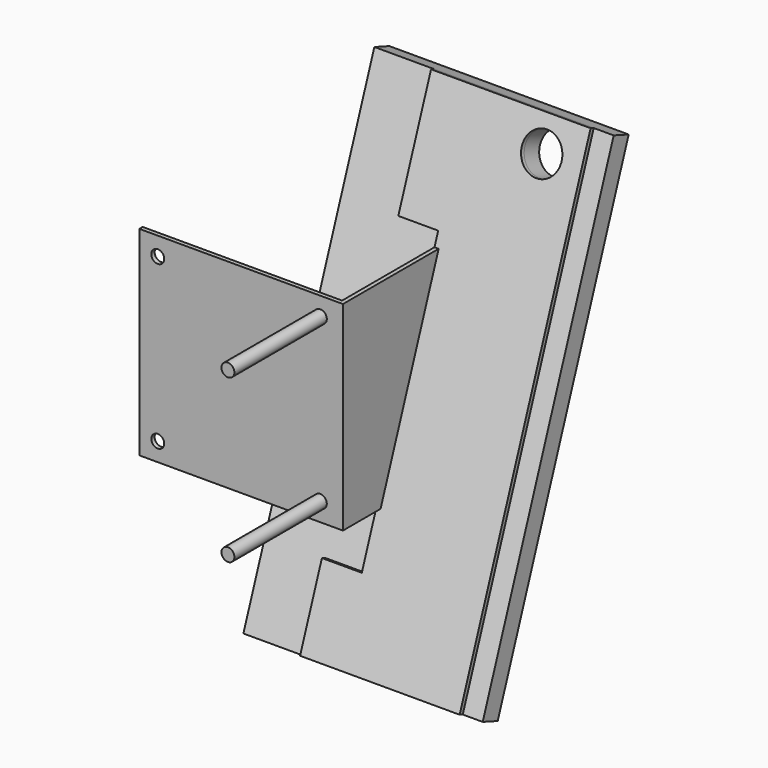
from build123d import *

# Parameters (mm, degrees)
F0_R      = 4.1275
F1_DEPTH  = 2.65684
F4_DEPTH  = 2.65684
F5_R      = 6.35
F5_R_2    = 4.1275
F6_DEPTH  = 6.35
F7_DEPTH  = 76.2
F8_R      = 12.7
F8_W      = 25.4
F8_H      = 76.2
F8_H_2    = 50.8
F9_DEPTH  = 2.65684
F10_W     = 152.4
F10_H     = 304.8
F10_R     = 12.7
F11_DEPTH = 12.7


with BuildPart() as f1:
    # F0 (on Front) → F1 (new body)
    with BuildSketch(Plane.XZ):
        with BuildLine():
            Line((47.625, -47.625), (46.9269177812, -47.625))
            ThreePointArc((46.9269177812, -47.625), (49.5524939874, -57.7092166749), (58.1025, -51.7525))
            ThreePointArc((58.1025, -51.7525), (54.4088955842, -45.9848260754), (47.625, -46.9269177812))
            Line((47.625, -46.9269177812), (47.625, -47.625))
        make_face()
        with Locations((51.7525, -51.7525)):
            Circle(F0_R, mode=Mode.SUBTRACT)
        with BuildLine():
            Line((46.9269177812, 47.625), (0, 47.625))
            Line((0, 47.625), (0, -47.625))
            Line((0, -47.625), (46.9269177812, -47.625))
            ThreePointArc((46.9269177812, -47.625), (47.2623719395, -47.2623719395), (47.625, -46.9269177812))
            Line((47.625, -46.9269177812), (47.625, 46.9269177812))
            ThreePointArc((47.625, 46.9269177812), (47.2623719395, 47.2623719395), (46.9269177812, 47.625))
        make_face()
        with BuildLine():
            Line((63.5, 63.5), (0, 63.5))
            Line((0, 63.5), (0, 47.625))
            Line((0, 47.625), (46.9269177812, 47.625))
            ThreePointArc((46.9269177812, 47.625), (49.5524939874, 57.7092166749), (58.1025, 51.7525))
            ThreePointArc((58.1025, 51.7525), (54.4088955842, 45.9848260754), (47.625, 46.9269177812))
            Line((47.625, 46.9269177812), (47.625, -46.9269177812))
            ThreePointArc((47.625, -46.9269177812), (54.4088955842, -45.9848260754), (58.1025, -51.7525))
            ThreePointArc((58.1025, -51.7525), (49.5524939874, -57.7092166749), (46.9269177812, -47.625))
            Line((46.9269177812, -47.625), (0, -47.625))
            Line((0, -47.625), (0, -63.5))
            Line((0, -63.5), (63.5, -63.5))
            Line((63.5, -63.5), (63.5, 63.5))
        make_face()
        with BuildLine():
            ThreePointArc((58.1025, 51.7525), (49.5524939874, 57.7092166749), (46.9269177812, 47.625))
            Line((46.9269177812, 47.625), (47.625, 47.625))
            Line((47.625, 47.625), (47.625, 46.9269177812))
            ThreePointArc((47.625, 46.9269177812), (54.4088955842, 45.9848260754), (58.1025, 51.7525))
        make_face()
        with Locations((51.7525, 51.7525)):
            Circle(F0_R, mode=Mode.SUBTRACT)
        with BuildLine():
            Line((47.625, 47.625), (46.9269177812, 47.625))
            ThreePointArc((46.9269177812, 47.625), (47.2623719395, 47.2623719395), (47.625, 46.9269177812))
            Line((47.625, 46.9269177812), (47.625, 47.625))
        make_face()
        with BuildLine():
            ThreePointArc((47.625, -46.9269177812), (47.2623719395, -47.2623719395), (46.9269177812, -47.625))
            Line((46.9269177812, -47.625), (47.625, -47.625))
            Line((47.625, -47.625), (47.625, -46.9269177812))
        make_face()
    extrude(amount=F1_DEPTH)

    # F2: F1 across plane


with BuildPart() as f1_1:
    add(f1.part)
    add(f1.part.mirror(Plane.YZ))

    # F3 (on face) → F4 (join)
    with BuildSketch(Plane.YZ.offset(63.5)):
        Polygon((-2.65684, 63.5), (-2.65684, -63.5), (27.3189402482, -63.5), (73.54316, 63.5), align=None)
    extrude(amount=F4_DEPTH)

    # F8 (on face) + F5 (on face) → F9 (join)
    with BuildSketch(Plane(origin=(0, 44.5317379162, -16.2082270816), x_dir=(-1, 0, 0), z_dir=(0, 0.9396926208, -0.3420201433))):
        Polygon((-63.5, 169.6484349915), (-139.7, 169.6484349915), (-139.7, -135.1515650085), (-63.5, -135.1515650085), (-63.5, -84.3515650085), (-63.5, 93.4484349915), align=None)
        with Locations((-114.3, 148.6934349915)):
            Circle(F8_R, mode=Mode.SUBTRACT)
        with Locations((-50.8, 131.5484349915)):
            Rectangle(F8_W, F8_H)
        with Locations((-50.8, -109.7515650085)):
            Rectangle(F8_W, F8_H_2)
    with BuildSketch(Plane(origin=(0, 0, 0), x_dir=(-1, 0, 0), z_dir=(0, 1, 0))):
        with Locations((-51.7525, 51.7525)):
            Circle(F5_R)
        with Locations((-51.7525, -51.7525)):
            Circle(F5_R)
    extrude(amount=F9_DEPTH, dir=(0, 0.9396926208, -0.3420201433))


with BuildPart() as f6:
    # F5 (on face) → F6 (new body)
    with BuildSketch(Plane(origin=(0, 0, 0), x_dir=(-1, 0, 0), z_dir=(0, 1, 0))):
        with Locations((-51.7525, 51.7525)):
            Circle(F5_R)
        with Locations((-51.7525, 51.7525)):
            Circle(F5_R_2, mode=Mode.SUBTRACT)
        with Locations((-51.7525, 51.7525)):
            Circle(F5_R_2)
    extrude(amount=F6_DEPTH)

    # F5 (on face) → F7, piece 2 (join)
    with BuildSketch(Plane(origin=(0, 0, 0), x_dir=(-1, 0, 0), z_dir=(0, 1, 0))):
        with Locations((-51.7525, 51.7525)):
            Circle(F5_R_2)
    extrude(amount=-F7_DEPTH)


with BuildPart() as f6b:
    # F5 (on face) → F6, piece 2 (new body)
    with BuildSketch(Plane(origin=(0, 0, 0), x_dir=(-1, 0, 0), z_dir=(0, 1, 0))):
        with Locations((-51.7525, -51.7525)):
            Circle(F5_R)
        with Locations((-51.7525, -51.7525)):
            Circle(F5_R_2, mode=Mode.SUBTRACT)
        with Locations((-51.7525, -51.7525)):
            Circle(F5_R_2)
    extrude(amount=F6_DEPTH)

    # F5 (on face) → F7 (join)
    with BuildSketch(Plane(origin=(0, 0, 0), x_dir=(-1, 0, 0), z_dir=(0, 1, 0))):
        with Locations((-51.7525, -51.7525)):
            Circle(F5_R_2)
    extrude(amount=-F7_DEPTH)


with BuildPart() as f11:
    # F10 (on face) → F11 (new body)
    with BuildSketch(Plane(origin=(0, 47.0283508588, -17.1169198792), x_dir=(-1, 0, 0), z_dir=(0, 0.9396926208, -0.3420201433))):
        with Locations((-76.2, 17.2484349915)):
            Rectangle(F10_W, F10_H)
        with Locations((-114.3, 148.6934349915)):
            Circle(F10_R, mode=Mode.SUBTRACT)
    extrude(amount=F11_DEPTH)


solid = Compound([f1_1.part, f6.part, f6b.part, f11.part])
